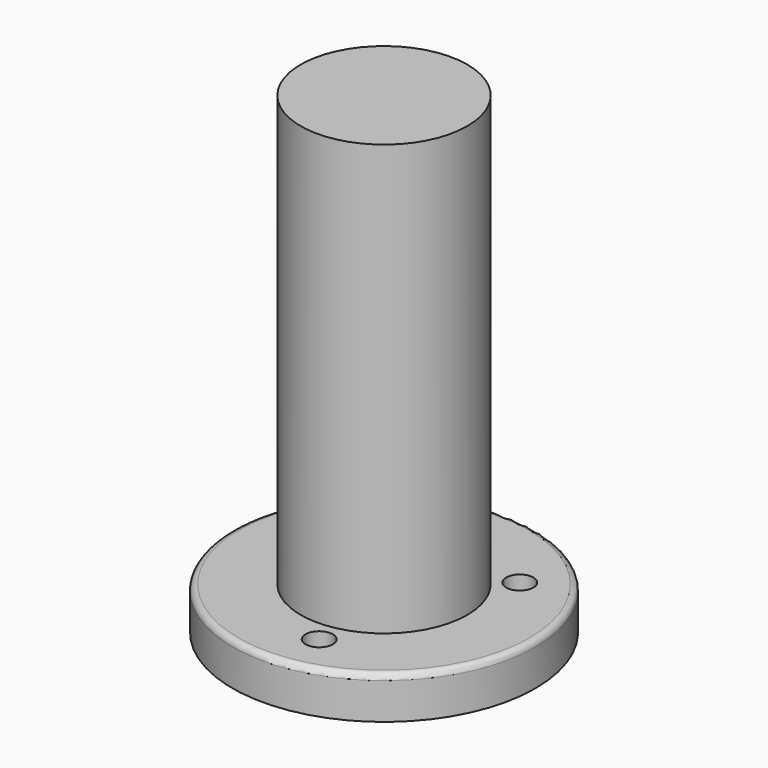
from build123d import *

# Parameters (mm, degrees)
F0_R           = 25
F0_R_2         = 13.75
F1_DEPTH       = 7
F2_DEPTH       = 78
F3_D           = 4.5
F3_CBORE_D     = 8.25
F3_CBORE_DEPTH = 4.5
F4_R           = 1


with BuildPart() as f1:
    # F0 (on Top) → F1 (new body)
    with BuildSketch(Plane.XY):
        Circle(F0_R)
        Circle(F0_R_2, mode=Mode.SUBTRACT)
    extrude(amount=F1_DEPTH)

    # F0 (on Top) → F2 (join)
    with BuildSketch(Plane.XY):
        Circle(F0_R_2)
    extrude(amount=F2_DEPTH)

    # F3 (through all)
    with Locations(Plane(origin=(0, 0, 0), x_dir=(1, 0, 0), z_dir=(0, 0, -1))):
        with Locations((3.0853754045, 17.2258659757), (13.3753498349, -11.2849464684), (-16.4607252394, -5.9409195073)):
            CounterBoreHole(F3_D / 2, F3_CBORE_D / 2, F3_CBORE_DEPTH)

    # F4
    f4_edges = [f1.edges().sort_by_distance(p)[0] for p in [
        (-25, 0, 7),
    ]]
    fillet(f4_edges, radius=F4_R)


solid = f1.part
